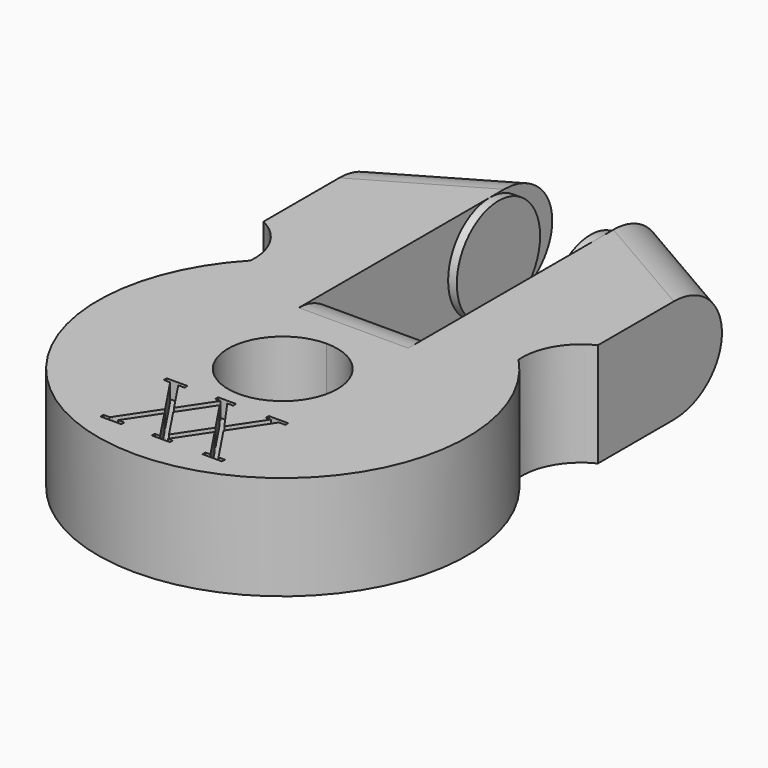
from build123d import *

# Parameters (mm, degrees)
F1_DEPTH = 6
F2_R     = 3
F3_DEPTH = 0.5
F4_R     = 3
F5_DEPTH = 0.5
F6_R     = 2.99999
F7_R     = 2.99999
F9_DEPTH = 1
F10_R    = 3
F11_R    = 2.99999


# Not quite as in the source:
# - a fillet or chamfer is up to 0.001 mm smaller than in the source, because OpenCascade refuses the exact size


with BuildPart() as f1:
    # F0 (on Top) → F1 (new body)
    with BuildSketch(Plane.XY):
        with BuildLine():
            Line((-3.15, 8.1), (-3.15, 10.1734949747))
            ThreePointArc((-3.15, 10.1734949747), (-5.6194604457, 9.046776459), (-7.7238904562, 7.3323949854))
            ThreePointArc((-7.7238904562, 7.3323949854), (0, -10.65), (7.7238904562, 7.3323949854))
            ThreePointArc((7.7238904562, 7.3323949854), (5.6194604457, 9.046776459), (3.15, 10.1734949747))
            Line((3.15, 10.1734949747), (3.15, 8.1))
            Line((3.15, 8.1), (0, 8.1))
            Line((0, 8.1), (-3.15, 8.1))
        make_face()
        with BuildLine():
            ThreePointArc((3.15, 0), (-2.2273863607, -2.2273863607), (0, 3.15))
            ThreePointArc((0, 3.15), (2.2273863607, 2.2273863607), (3.15, 0))
        make_face(mode=Mode.SUBTRACT)
        with BuildLine():
            ThreePointArc((-7.7238904562, 7.3323949854), (-5.6194604457, 9.046776459), (-3.15, 10.1734949747))
            Line((-3.15, 10.1734949747), (-3.15, 23.35))
            Line((-3.15, 23.35), (-9.6377339195, 19.5871143267))
            Line((-9.6377339195, 19.5871143267), (-9.6377339195, 10.6575252249))
            ThreePointArc((-9.6377339195, 10.6575252249), (-8.1670066914, 9.2906908645), (-7.7238904562, 7.3323949854))
        make_face()
        with BuildLine():
            ThreePointArc((3.15, 10.1734949747), (5.6194604457, 9.046776459), (7.7238904562, 7.3323949854))
            ThreePointArc((7.7238904562, 7.3323949854), (8.1670066914, 9.2906908645), (9.6377339195, 10.6575252249))
            Line((9.6377339195, 10.6575252249), (9.6377339195, 19.5871143267))
            Line((9.6377339195, 19.5871143267), (3.15, 23.35))
            Line((3.15, 23.35), (3.15, 10.1734949747))
        make_face()
    extrude(amount=F1_DEPTH)

    # F2 (on face) → F3 (join)
    with BuildSketch(Plane.YZ.offset(-3.15)):
        with Locations((18.85, 3)):
            Circle(F2_R)
    extrude(amount=F3_DEPTH)

    # F4 (on face) → F5 (join)
    with BuildSketch(Plane(origin=(3.15, 0, 0), x_dir=(0, -1, 0), z_dir=(-1, 0, 0))):
        with Locations((-18.85, 3)):
            Circle(F4_R)
    extrude(amount=F5_DEPTH)

    # F6 (radius 3 in the source; OpenCascade refuses exactly that, so slightly less here)
    f6_edges = [f1.edges().sort_by_distance(p)[0] for p in [
        (-6.393867, 21.468557, 0),
        (-6.393867, 21.468557, 6),
    ]]
    fillet(f6_edges, radius=F6_R)

    # F7 (radius 3 in the source; OpenCascade refuses exactly that, so slightly less here)
    f7_edges = [f1.edges().sort_by_distance(p)[0] for p in [
        (6.393867, 21.468557, 0),
        (6.393867, 21.468557, 6),
    ]]
    fillet(f7_edges, radius=F7_R)

    # F8 (on face) → F9 (cut)
    with BuildSketch(Plane.XY.offset(6)):
        Polygon((-0.5410675658, -4.1934514275), (-0.2322952287, -4.1934514275), (-1.4496098506, -6.0194233604), (-2.6669244725, -4.1934514275), (-2.3, -4.1934514275), (-2.3, -3.9827399887), (-3.5, -3.9827399887), (-3.5, -4.1934514275), (-3.1341812573, -4.1934514275), (-2.8992197012, -4.5418942706), (-1.6819050793, -6.3678662034), (-3.0600394749, -8.4350677969), (-3.1399389263, -8.5422809794), (-3.5, -8.5422809794), (-3.5, -8.7529924182), (-2.3, -8.7529924182), (-2.3, -8.5422809794), (-2.6669244725, -8.5422809794), (-1.4496098506, -6.7163090465), (-0.2322952287, -8.5422809794), (-0.5410675658, -8.5422809794), (-0.5410675658, -8.7529924182), (0.5013382179, -8.7529924182), (0.5013382179, -8.5422809794), (0.2322952287, -8.5422809794), (1.4496098506, -6.7163090465), (2.6669244725, -8.5422809794), (2.3810260464, -8.5422809794), (2.3810260464, -8.7529924182), (3.4986780956, -8.7529924182), (3.5, -8.5422809794), (3.1424169429, -8.5422809794), (3.0600394749, -8.4350677969), (1.6819050793, -6.3678662034), (2.8992197012, -4.5418942706), (3.1315149299, -4.1934514275), (3.3579636365, -4.1934514275), (3.5, -4.1934514275), (3.4986780956, -3.9827399887), (2.3810260464, -3.9827399887), (2.3810260464, -4.1934514275), (2.6669244725, -4.1934514275), (1.4496098506, -6.0194233604), (0.1581401168, -4.1934514275), (0.5013382179, -4.1934514275), (0.5013382179, -3.9827399887), (-0.5410675658, -3.9827399887), align=None)
        Polygon((-1.2173146219, -6.3678662034), (0, -4.5418942706), (1.2173146219, -6.3678662034), (0, -8.1938381363), align=None, mode=Mode.SUBTRACT)
    extrude(amount=-F9_DEPTH, mode=Mode.SUBTRACT)

    # F10
    f10_edges = [f1.edges().sort_by_distance(p)[0] for p in [
        (0, 8.1, 6),
    ]]
    fillet(f10_edges, radius=F10_R)

    # F11 (radius 3 in the source; OpenCascade refuses exactly that, so slightly less here)
    f11_edges = [f1.edges().sort_by_distance(p)[0] for p in [
        (0, 8.1, 0),
    ]]
    fillet(f11_edges, radius=F11_R)


solid = f1.part
